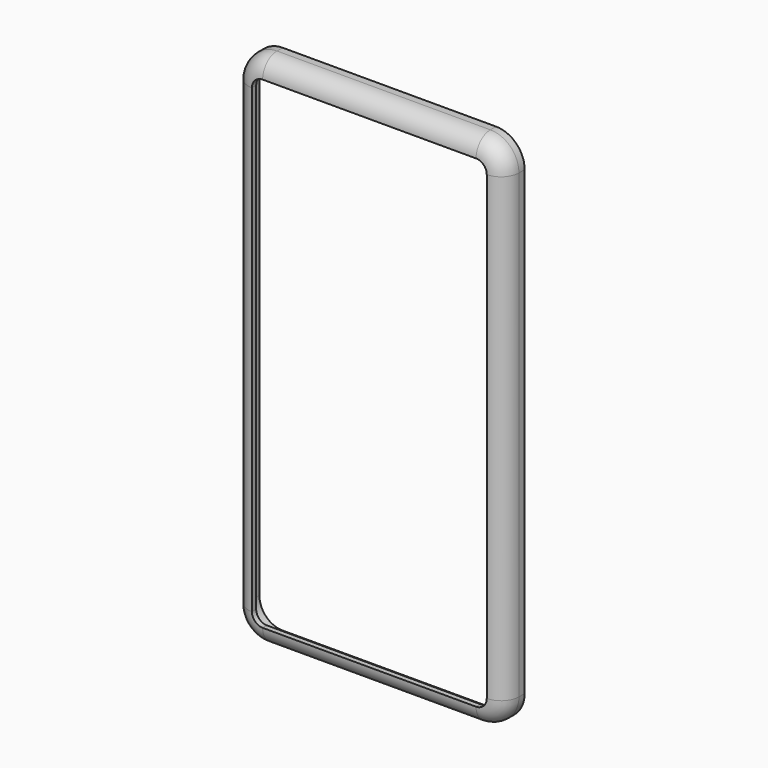
from build123d import *

# Parameters (mm, degrees)
F1_DEPTH = 5.11
F2_R     = 5
F3_DEPTH = 7
F4_R     = 5
F5_T     = -1.5


# Not quite as in the source:
# - a shell that OpenCascade refuses in one call is made with other operations: the cavity is built on its own and cut out


with BuildPart() as f1:
    # F0 (on Front) → F1 (new body)
    with BuildSketch(Plane.XZ):
        with BuildLine():
            Line((28.845, 71.765), (-28.845, 71.765))
            ThreePointArc((-28.845, 71.765), (-34.5018542495, 69.4218542495), (-36.845, 63.765))
            Line((-36.845, 63.765), (-36.845, -63.765))
            ThreePointArc((-36.845, -63.765), (-34.5018542495, -69.4218542495), (-28.845, -71.765))
            Line((-28.845, -71.765), (28.845, -71.765))
            ThreePointArc((28.845, -71.765), (34.5018542495, -69.4218542495), (36.845, -63.765))
            Line((36.845, -63.765), (36.845, 63.765))
            ThreePointArc((36.845, 63.765), (34.5018542495, 69.4218542495), (28.845, 71.765))
        make_face()
    extrude(amount=F1_DEPTH)

    # F2
    f2_edges = [f1.edges().sort_by_distance(p)[0] for p in [
        (36.845, -5.11, 0),
    ]]
    fillet(f2_edges, radius=F2_R)

    # F0 (on Front) → F3 (join)
    with BuildSketch(Plane.XZ):
        with BuildLine():
            Line((29.845, 72.5), (-29.845, 72.5))
            ThreePointArc((-29.845, 72.5), (-35.5018542495, 70.1568542495), (-37.845, 64.5))
            Line((-37.845, 64.5), (-37.845, -64.5))
            ThreePointArc((-37.845, -64.5), (-35.5018542495, -70.1568542495), (-29.845, -72.5))
            Line((-29.845, -72.5), (29.845, -72.5))
            ThreePointArc((29.845, -72.5), (35.5018542495, -70.1568542495), (37.845, -64.5))
            Line((37.845, -64.5), (37.845, 64.5))
            ThreePointArc((37.845, 64.5), (35.5018542495, 70.1568542495), (29.845, 72.5))
        make_face()
        with BuildLine():
            ThreePointArc((-36.845, 63.765), (-34.5018542495, 69.4218542495), (-28.845, 71.765))
            Line((-28.845, 71.765), (28.845, 71.765))
            ThreePointArc((28.845, 71.765), (34.5018542495, 69.4218542495), (36.845, 63.765))
            Line((36.845, 63.765), (36.845, -63.765))
            ThreePointArc((36.845, -63.765), (34.5018542495, -69.4218542495), (28.845, -71.765))
            Line((28.845, -71.765), (-28.845, -71.765))
            ThreePointArc((-28.845, -71.765), (-34.5018542495, -69.4218542495), (-36.845, -63.765))
            Line((-36.845, -63.765), (-36.845, 63.765))
        make_face(mode=Mode.SUBTRACT)
        with BuildLine():
            Line((28.845, 71.765), (-28.845, 71.765))
            ThreePointArc((-28.845, 71.765), (-34.5018542495, 69.4218542495), (-36.845, 63.765))
            Line((-36.845, 63.765), (-36.845, -63.765))
            ThreePointArc((-36.845, -63.765), (-34.5018542495, -69.4218542495), (-28.845, -71.765))
            Line((-28.845, -71.765), (28.845, -71.765))
            ThreePointArc((28.845, -71.765), (34.5018542495, -69.4218542495), (36.845, -63.765))
            Line((36.845, -63.765), (36.845, 63.765))
            ThreePointArc((36.845, 63.765), (34.5018542495, 69.4218542495), (28.845, 71.765))
        make_face()
    extrude(amount=F3_DEPTH)

    # F4
    f4_edges = [f1.edges().sort_by_distance(p)[0] for p in [
        (37.845, -7, 0),
    ]]
    fillet(f4_edges, radius=F4_R)

    # F5: a shell. OpenCascade refuses it in one call, so the cavity is built on its own and cut out:
    # the body offset inwards by the wall thickness, plus a prism from it out through each open face.
    f5_core = offset(f1.part, amount=F5_T, kind=Kind.INTERSECTION, mode=Mode.PRIVATE)
    f5_exits = [f5_core.faces().sort_by_distance(p)[0] for p in [
        (0, -1.5, 0),
        (0, -5.5, 0),
    ]]
    add(f5_core, mode=Mode.SUBTRACT)
    extrude(f5_exits, amount=-F5_T, mode=Mode.SUBTRACT)


solid = f1.part
